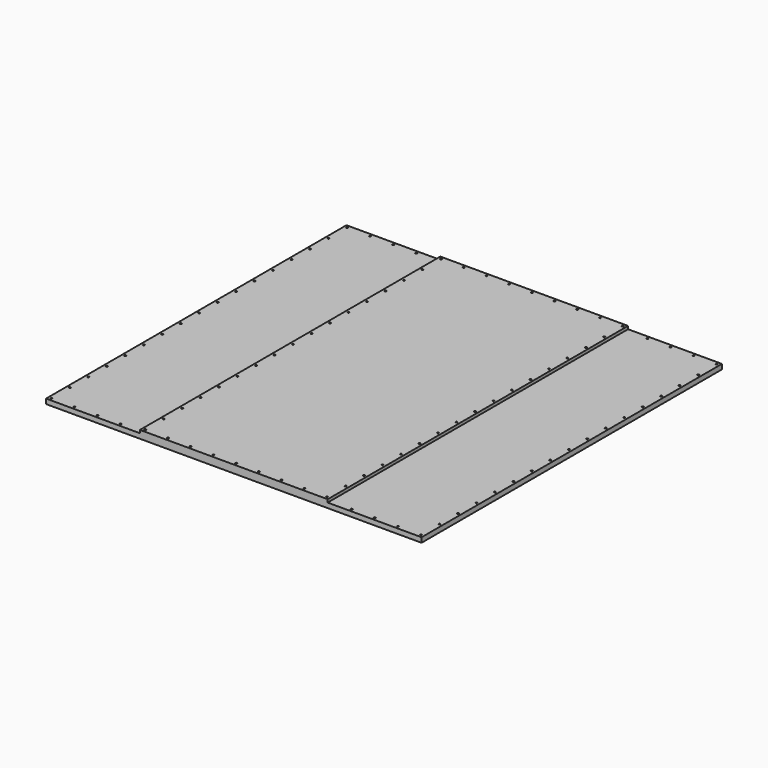
from build123d import *

# Parameters (mm, degrees)
F0_W            = 1219.2
F0_H            = 1219.2
F1_DEPTH        = 15.875
F2_W            = 1219.2
F2_H            = 2438.4
F3_DEPTH        = 15.875
F4_W            = 2438.4
F4_H            = 1219.2
F5_DEPTH        = 15.875
F6_W            = 2438.4
F6_H            = 1219.2
F7_DEPTH        = 15.875
F9_D            = 5
F9_CSINK_D      = 11.2
F9_CSINK_ANGLE  = 90
F11_DEPTH       = 19.05
F13_D           = 5
F13_CSINK_D     = 11.2
F13_CSINK_ANGLE = 90


# Not quite as in the source:
# - a length typed as a fraction of an inch, garbled in the dataset ("3 / 203.2 mm" for 3/8 in), is restored


with BuildPart() as f1:
    # F0 (on Top) → F1 (new body)
    with BuildSketch(Plane.XY):
        with Locations((609.6, 609.6)):
            Rectangle(F0_W, F0_H)
        with Locations((609.6, -609.6)):
            Rectangle(F0_W, F0_H)
    extrude(amount=F1_DEPTH)

    # F2 (on Top) → F3 (join)
    with BuildSketch(Plane.XY):
        with Locations((-609.6, 0)):
            Rectangle(F2_W, F2_H)
    extrude(amount=F3_DEPTH)

    # F4 (on face) → F5 (join)
    with BuildSketch(Plane(origin=(0, 0, 0), x_dir=(1, 0, 0), z_dir=(0, 0, -1))):
        with Locations((0, -609.6)):
            Rectangle(F4_W, F4_H)
    extrude(amount=F5_DEPTH)

    # F6 (on face) → F7 (join)
    with BuildSketch(Plane(origin=(0, 0, 0), x_dir=(1, 0, 0), z_dir=(0, 0, -1))):
        with Locations((0, 609.6)):
            Rectangle(F6_W, F6_H)
    extrude(amount=F7_DEPTH)

    # F9 (through all)
    with Locations(Plane.XY.offset(15.875)):
        with Locations((-1200.15, 600.075), (-1200.15, 450.05625), (-1200.15, 300.0375), (-1200.15, 150.01875), (-1200.15, 0), (-1200.15, -150.01875), (-1200.15, -300.0375), (-1200.15, -450.05625), (-1200.15, -600.075), (-1200.15, -750.09375), (-1200.15, -900.1125), (-1200.15, -1050.13125), (-1200.15, -1200.15), (-1050.13125, -1200.15), (-900.1125, -1200.15), (-750.09375, -1200.15), (-600.075, -1200.15), (-450.05625, -1200.15), (-300.0375, -1200.15), (-150.01875, -1200.15), (-1200.15, 750.09375), (-1200.15, 900.1125), (-1200.15, 1050.13125), (-1200.15, 1200.15), (-1050.13125, 1200.15), (-900.1125, 1200.15), (-750.09375, 1200.15), (-600.075, 1200.15), (-450.05625, 1200.15), (-300.0375, 1200.15), (-150.01875, 1200.15), (0, 1200.15), (150.01875, 1200.15), (300.0375, 1200.15), (450.05625, 1200.15), (600.075, 1200.15), (750.09375, 1200.15), (900.1125, 1200.15), (1050.13125, 1200.15), (1200.15, 1200.15), (1200.15, 1050.13125), (1200.15, 900.1125), (1200.15, 750.09375), (1200.15, 600.075), (1200.15, 450.05625), (1200.15, 300.0375), (1200.15, 150.01875), (1200.15, 0), (1200.15, -150.01875), (1200.15, -300.0375), (1200.15, -450.05625), (1200.15, -600.075), (1200.15, -750.09375), (1200.15, -900.1125), (1200.15, -1050.13125), (1200.15, -1200.15), (1050.13125, -1200.15), (900.1125, -1200.15), (750.09375, -1200.15), (600.075, -1200.15), (450.05625, -1200.15), (300.0375, -1200.15), (150.01875, -1200.15), (0, -1200.15), (0, -1200.15), (150.01875, -1200.15), (300.0375, -1200.15), (450.05625, -1200.15), (600.075, -1200.15), (750.09375, -1200.15), (900.1125, -1200.15)):
            CounterSinkHole(F9_D / 2, F9_CSINK_D / 2, counter_sink_angle=F9_CSINK_ANGLE)

    # F10 (on face) → F11 (join)
    with BuildSketch(Plane.XY.offset(15.875)):
        Polygon((0, 1219.2), (-609.6, 1219.2), (-609.6, -1219.2), (609.6, -1219.2), (609.6, 1219.2), align=None)
    extrude(amount=F11_DEPTH)

    # F13 (through all)
    with Locations(Plane.XY.offset(34.925)):
        with Locations((-590.55, 1200.15), (-442.9125, 1200.15), (-295.275, 1200.15), (-147.6375, 1200.15), (0, 1200.15), (147.6375, 1200.15), (295.275, 1200.15), (442.9125, 1200.15), (590.55, 1050.13125), (590.55, 1200.15), (590.55, 900.1125), (590.55, 750.09375), (590.55, 600.075), (590.55, 450.05625), (590.55, 300.0375), (590.55, 150.01875), (590.55, 0), (590.55, -150.01875), (590.55, -300.0375), (590.55, -450.05625), (590.55, -600.075), (590.55, -750.09375), (590.55, -900.1125), (590.55, -1050.13125), (590.55, -1200.15), (442.9125, -1200.15), (295.275, -1200.15), (147.6375, -1200.15), (0, -1200.15), (-147.6375, -1200.15), (-295.275, -1200.15), (-442.9125, -1200.15), (-590.55, -1200.15), (-590.55, -1050.13125), (-590.55, -900.1125), (-590.55, -750.09375), (-590.55, -600.075), (-590.55, -450.05625), (-590.55, -300.0375), (-590.55, -150.01875), (-590.55, 0), (-590.55, 150.01875), (-590.55, 300.0375), (-590.55, 450.05625), (-590.55, 600.075), (-590.55, 750.09375), (-590.55, 900.1125), (-590.55, 1050.13125), (-590.55, -750.09375), (-590.55, -600.075), (-590.55, -450.05625), (-590.55, -300.0375), (-590.55, -150.01875), (-590.55, 0), (-590.55, 150.01875), (-590.55, 300.0375), (-590.55, 450.05625), (-590.55, 600.075), (-590.55, 750.09375), (-590.55, 900.1125), (-590.55, 1050.13125)):
            CounterSinkHole(F13_D / 2, F13_CSINK_D / 2, counter_sink_angle=F13_CSINK_ANGLE)


solid = f1.part
